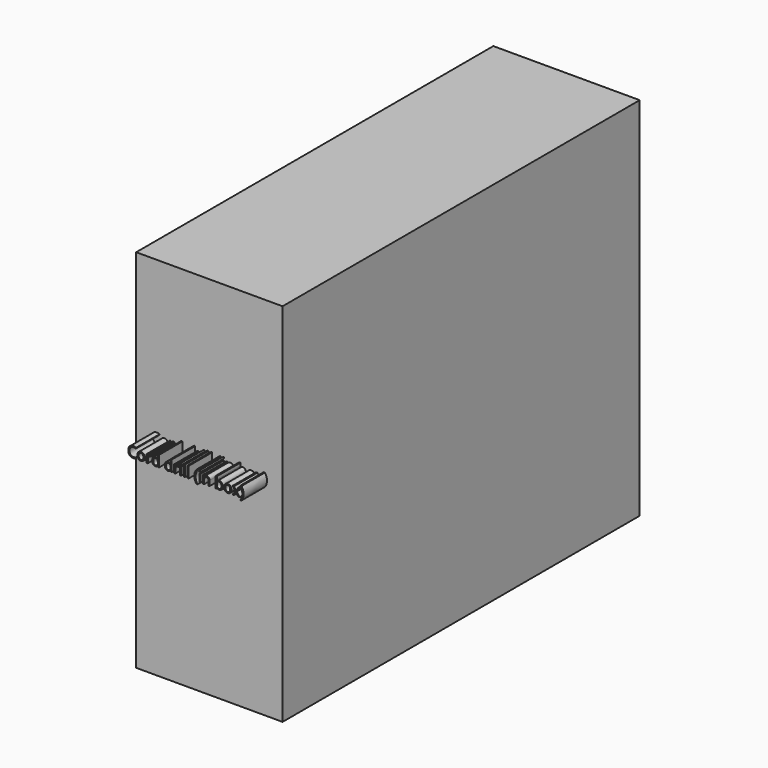
from build123d import *

# Parameters (mm, degrees)
F0_W         = 127
F0_H         = 317.5
F1_DEPTH     = 387.35
F2_TEXT_SIZE = 12.6370615101
F3_DEPTH     = 25.4


# Not quite as in the source:
# - Text() gives the source's letters only with a copy of the font that has no kerning and outlines rounded to 1/6400 em; it was checked with that copy


with BuildPart() as f1:
    # F0 (on Front) → F1 (new body)
    with BuildSketch(Plane.XZ):
        Rectangle(F0_W, F0_H)
    extrude(amount=F1_DEPTH)

    # F2 (on face) → F3 (join)
    with BuildSketch(Plane.XZ.offset(387.35)):
        with Locations((-50.8, 17.6898964231)):
            Text('Cord drill (in box)', F2_TEXT_SIZE, font='Open Sans', text_align=(TextAlign.LEFT, TextAlign.BOTTOM))
    extrude(amount=F3_DEPTH)


solid = f1.part
